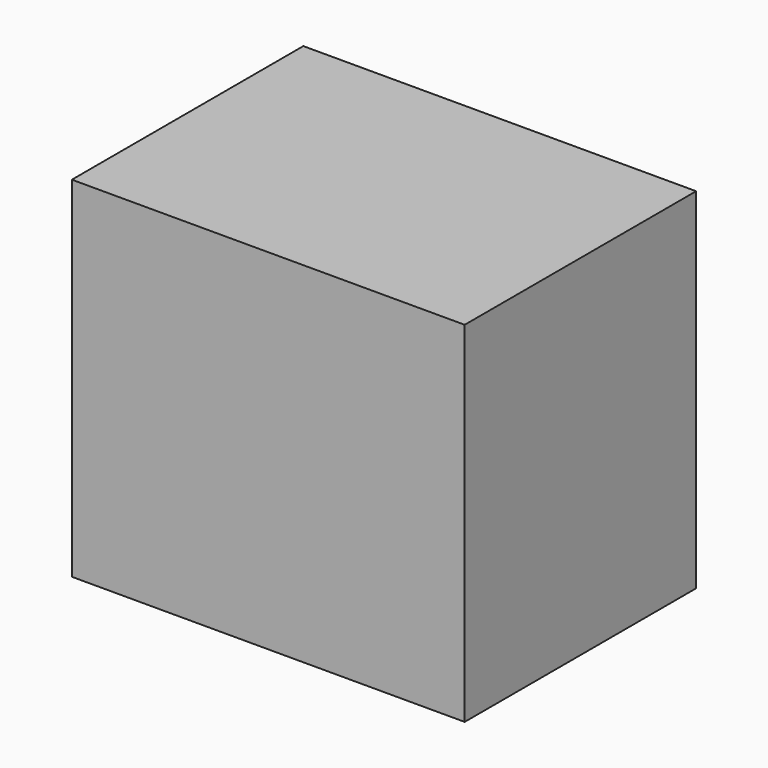
from build123d import *

# Parameters (mm, degrees)
F0_W     = 100
F0_H     = 73.6472510436
F1_DEPTH = 89


# Not quite as in the source:
# - the program builds the solid bodies; features that only make, move or delete a surface that nothing else refers to are left out


with BuildPart() as f1:
    # F0 (on Top) → F1 (new body)
    with BuildSketch(Plane.XY):
        Rectangle(F0_W, F0_H)
    extrude(amount=F1_DEPTH)


solid = f1.part
